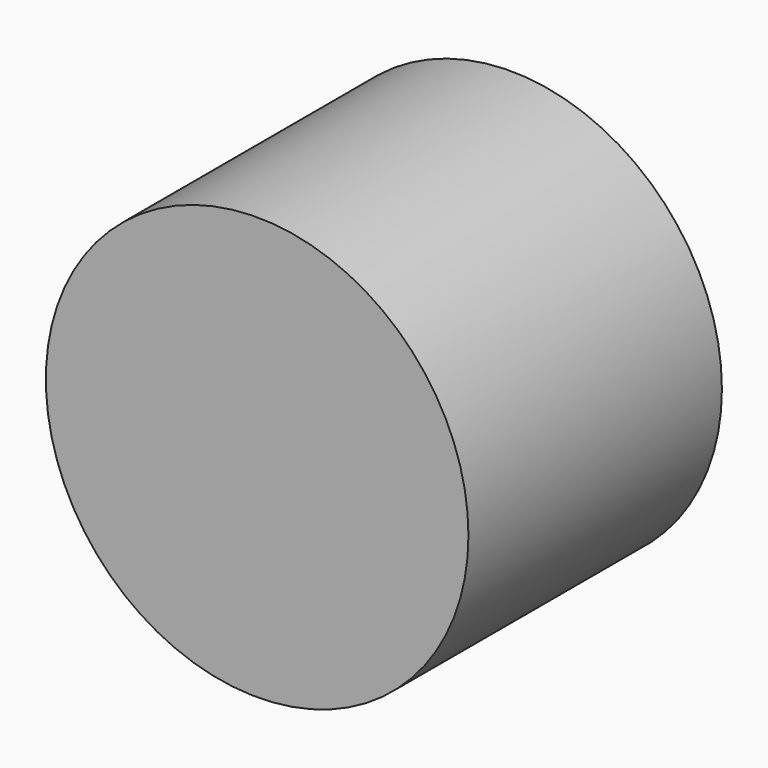
from build123d import *

# Parameters (mm, degrees)
F0_R     = 33.3435251751
F1_DEPTH = 50


# Not quite as in the source:
# - the program builds the solid bodies; features that only make, move or delete a surface that nothing else refers to are left out


with BuildPart() as f1:
    # F0 (on Front) → F1 (new body)
    with BuildSketch(Plane.XZ):
        with Locations((-29.3218102306, 27.88564004)):
            Circle(F0_R)
    extrude(amount=F1_DEPTH)


solid = f1.part
